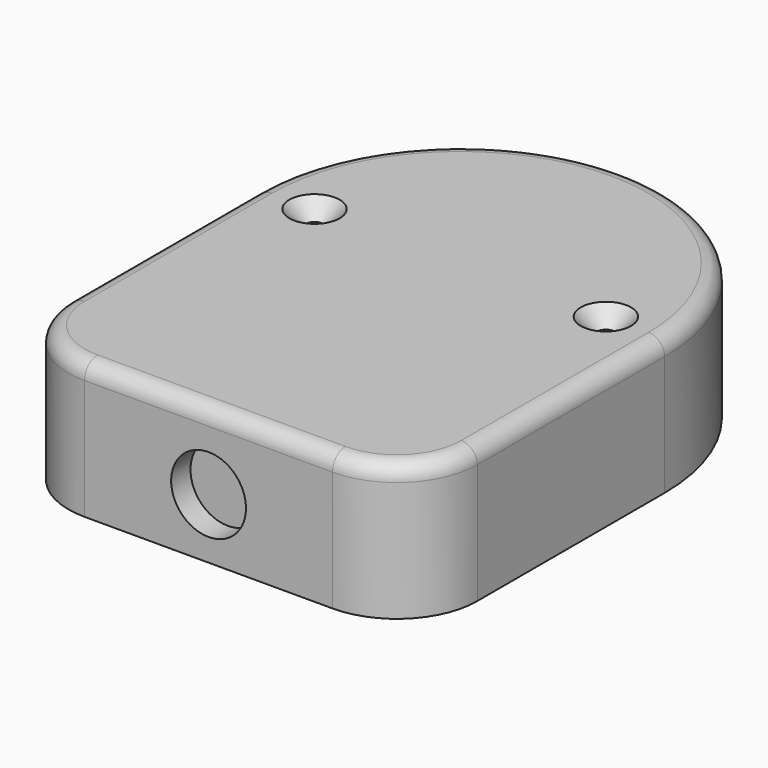
from build123d import *

# Parameters (mm, degrees)
F1_R      = 7.62
F2_DEPTH  = 8.9916
F3_R      = 3.175
F4_DEPTH  = 18.5
F7_DEPTH  = 21.5
F5_R      = 1.4351
F8_DEPTH  = 25.4
F11_DEPTH = 20
F12_R     = 2.54
F13_SIZE  = 2.54
F6_R      = 30.2514
F14_DEPTH = 2.032
F16_R     = 30.2514
F17_DEPTH = 2.032
F18_R     = 5.9079449729
F19_DEPTH = 3.81
F20_R     = 3.175
F20_R_2   = 1.016
F21_DEPTH = 20


# Not quite as in the source:
# - a feature of the source that left no trace in its solid (it failed there, or was rolled back) is left out
# - a feature names something its author has since deleted; it is built from what else it names


with BuildPart() as f2:
    # F1 (on Top) → F2 (new body)
    with BuildSketch(Plane.XY):
        with BuildLine():
            Line((14.3891, -27.8892), (14.3891, 5.7461149649))
            ThreePointArc((14.3891, 5.7461149649), (0, 15.494), (-14.3891, 5.7461149649))
            Line((-14.3891, 5.7461149649), (-14.3891, -27.8892))
            Line((-14.3891, -27.8892), (14.3891, -27.8892))
        make_face()
        Circle(F1_R, mode=Mode.SUBTRACT)
    extrude(amount=F2_DEPTH)


with BuildPart() as f4:
    # F3 (on Top) → F4 (new body)
    with BuildSketch(Plane.XY):
        Circle(F3_R)
    extrude(amount=F4_DEPTH)


with BuildPart() as f7:
    # F0 (on Top) → F7 (new body)
    with BuildSketch(Plane.XY):
        with BuildLine():
            Line((32.2834, -36.9807843447), (32.2834, 0))
            ThreePointArc((32.2834, 0), (0, 32.2834), (-32.2834, 0))
            Line((-32.2834, 0), (-32.2834, -36.9807843447))
            ThreePointArc((-32.2834, -36.9807843447), (-28.5636561211, -45.9610404657), (-19.5834, -49.6807843447))
            Line((-19.5834, -49.6807843447), (19.5834, -49.6807843447))
            ThreePointArc((19.5834, -49.6807843447), (28.5636561211, -45.9610404657), (32.2834, -36.9807843447))
        make_face()
    extrude(amount=F7_DEPTH)

    # F5 (on Top) → F8 (cut)
    with BuildSketch(Plane.XY):
        with Locations((-23.0124, 0)):
            Circle(F5_R)
        with Locations((23.0124, 0)):
            Circle(F5_R)
    extrude(amount=F8_DEPTH, mode=Mode.SUBTRACT)


with BuildPart() as f11_tool:
    # F10 (on Top) → F11 (new body)
    with BuildSketch(Plane.XY):
        with BuildLine():
            Line((-23.5020610966, -3.7882152164), (-27.6819982204, -3.7882152164))
            ThreePointArc((-27.6819982204, -3.7882152164), (-0.010778614, -27.9399979209), (27.6790671673, -3.8095722529))
            Line((27.6790671673, -3.8095722529), (23.0213215121, -3.8095722529))
            ThreePointArc((23.0213215121, -3.8095722529), (19.1556447136, -0.1037564295), (22.8138242261, 3.8070300236))
            ThreePointArc((22.8138242261, 3.8070300236), (22.9642316699, 3.81), (23.1146391137, 3.8070300236))
            Line((23.1146391137, 3.8070300236), (27.6794169447, 3.8070300236))
            ThreePointArc((27.6794169447, 3.8070300236), (-0.0092095477, 27.9399984822), (-27.6819206668, 3.7887818881))
            Line((-27.6819206668, 3.7887818881), (-23.4967496803, 3.7887818881))
            ThreePointArc((-23.4967496803, 3.7887818881), (-19.3067133937, 0.4041926109), (-22.688364657, -3.7882152164))
            ThreePointArc((-22.688364657, -3.7882152164), (-23.0952128768, -3.81), (-23.5020610966, -3.7882152164))
        make_face()
        with BuildLine():
            ThreePointArc((27.6790671673, -3.8095722529), (-0.010778614, -27.9399979209), (-27.6819982204, -3.7882152164))
            Line((-27.6819982204, -3.7882152164), (-27.6819982204, -34.7421456456))
            ThreePointArc((-27.6819982204, -34.7421456456), (-24.7062031172, -41.9263505425), (-17.5219982204, -44.9021456456))
            Line((-17.5219982204, -44.9021456456), (17.5190671673, -44.9021456456))
            ThreePointArc((17.5190671673, -44.9021456456), (24.7032720641, -41.9263505425), (27.6790671673, -34.7421456456))
            Line((27.6790671673, -34.7421456456), (27.6790671673, -3.8095722529))
        make_face()
        with BuildLine():
            Line((-22.688364657, -3.7882152164), (-23.5020610966, -3.7882152164))
            ThreePointArc((-23.5020610966, -3.7882152164), (-23.0952128768, -3.81), (-22.688364657, -3.7882152164))
        make_face()
        with BuildLine():
            ThreePointArc((23.1146391137, 3.8070300236), (22.9642316699, 3.81), (22.8138242261, 3.8070300236))
            Line((22.8138242261, 3.8070300236), (23.1146391137, 3.8070300236))
        make_face()
    extrude(amount=F11_DEPTH)


with BuildPart() as f2_1:
    add(f2.part)

    # F11: cut by f11_tool
    add(f11_tool.part, mode=Mode.SUBTRACT)


with BuildPart() as f4_1:
    add(f4.part)

    # F11: cut by f11_tool
    add(f11_tool.part, mode=Mode.SUBTRACT)


with BuildPart() as f7_1:
    add(f7.part)

    # F11: cut by f11_tool
    add(f11_tool.part, mode=Mode.SUBTRACT)

    # F12
    f12_edges = [f7_1.edges().sort_by_distance(p)[0] for p in [
        (0, 32.2834, 21.5),
        (32.2834, -18.490392, 21.5),
        (28.563656, -45.96104, 21.5),
        (0, -49.680784, 21.5),
        (-32.2834, -18.490392, 21.5),
        (-28.563656, -45.96104, 21.5),
    ]]
    fillet(f12_edges, radius=F12_R)

    # F13
    f13_edges = [f7_1.edges().sort_by_distance(p)[0] for p in [
        (-24.4475, 0, 21.5),
        (21.5773, 0, 21.5),
    ]]
    chamfer(f13_edges, length=F13_SIZE)

    # F6 (on Top) → F14 (cut)
    with BuildSketch(Plane.XY):
        Circle(F6_R)
    extrude(amount=F14_DEPTH, mode=Mode.SUBTRACT)

    # F16 (on Top) + F6 (on Top) → F17 (cut)
    with BuildSketch(Plane.XY):
        Circle(F16_R)
    with BuildSketch(Plane.XY):
        Circle(F6_R)
    extrude(amount=F17_DEPTH, mode=Mode.SUBTRACT)

    # F18 (on face) → F19 (cut)
    with BuildSketch(Plane.XZ.offset(49.6807843447)):
        with Locations((0, 9.48)):
            Circle(F18_R)
    extrude(amount=-F19_DEPTH, mode=Mode.SUBTRACT)

    # F20 (on face) → F21 (join, through all)
    with BuildSketch(Plane(origin=(0, 0, 20), x_dir=(1, 0, 0), z_dir=(0, 0, -1))):
        with Locations((17.5190671673, 34.7421456456)):
            Circle(F20_R)
        with Locations((17.5190671673, 34.7421456456)):
            Circle(F20_R_2, mode=Mode.SUBTRACT)
        with Locations((-17.5219982204, 34.7421456456)):
            Circle(F20_R)
        with Locations((-17.5219982204, 34.7421456456)):
            Circle(F20_R_2, mode=Mode.SUBTRACT)
    extrude(amount=F21_DEPTH)


solid = f7_1.part
